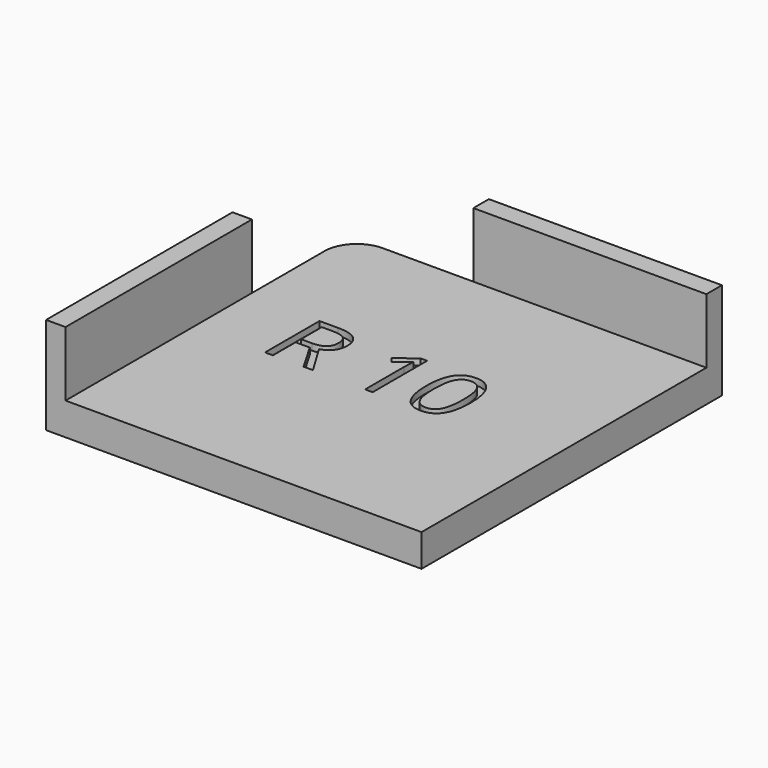
from build123d import *

# Parameters (mm, degrees)
F1_DEPTH      = 5
F2_W          = 3
F2_H          = 36
F2_W_2        = 36
F2_H_2        = 3
F3_DEPTH      = 10
F3_DEPTH_BACK = 5
F4_TEXT_SIZE  = 14.7307043118
F5_DEPTH      = 1


# Not quite as in the source:
# - Text() gives the source's letters only with a copy of the font that has no kerning and outlines rounded to 1/6400 em; it was checked with that copy


with BuildPart() as f1:
    # F0 (on Top) → F1 (new body)
    with BuildSketch(Plane.XY):
        with BuildLine():
            Line((50, 5), (0, 5))
            ThreePointArc((0, 5), (-3.5355339059, 3.5355339059), (-5, 0))
            Line((-5, 0), (-5, -50))
            Line((-5, -50), (50, -50))
            Line((50, -50), (50, 5))
        make_face()
    extrude(amount=F1_DEPTH)

    # F2 (on face) → F3 (join, two sides)
    with BuildSketch(Plane.XY.offset(5)) as f3_sk:
        with Locations((-6.5, -32)):
            Rectangle(F2_W, F2_H)
        with Locations((32, 6.5)):
            Rectangle(F2_W_2, F2_H_2)
    extrude(amount=F3_DEPTH)
    extrude(f3_sk.sketch, amount=-F3_DEPTH_BACK)

    # F4 (on face) → F5 (cut)
    with BuildSketch(Plane.XY.offset(5)):
        with Locations((4.4858261352, -25.144356166)):
            Text('R 10', F4_TEXT_SIZE, font='Open Sans', text_align=(TextAlign.LEFT, TextAlign.BOTTOM))
    extrude(amount=-F5_DEPTH, mode=Mode.SUBTRACT)


with BuildPart() as f6_1:
    # F6: copy of F1
    add(f1.part)


solid = f1.part
